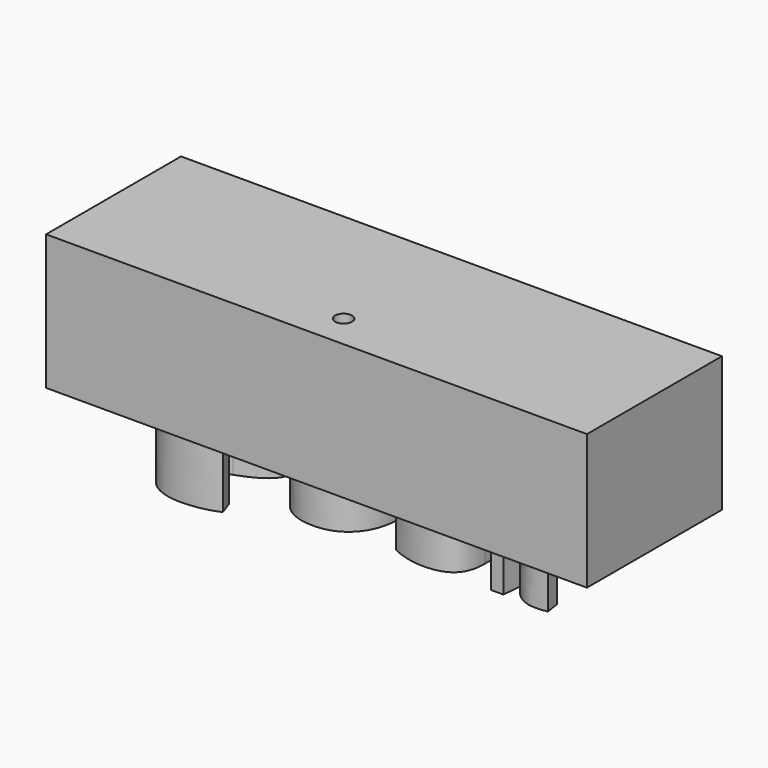
from build123d import *

# Parameters (mm, degrees)
F0_W         = 101.6
F0_H         = 31.6853369992
F1_DEPTH     = 12.7
F3_DEPTH     = 12.7
F5_DEPTH     = 59.182
F2_TEXT_SIZE = 35.1481081081
F6_DEPTH     = 12.7


# Not quite as in the source:
# - Text() gives the source's letters only with a copy of the font that has no kerning and outlines rounded to 1/6400 em; it was checked with that copy


with BuildPart() as f1:
    # F0 (on Top) → F1 (new body)
    with BuildSketch(Plane.XY):
        Rectangle(F0_W, F0_H)
    extrude(amount=F1_DEPTH)

    # F3 (add): a face of the model
    f3_faces = [f1.faces().sort_by_distance(p)[0] for p in [
        (0, 0, 12.7),
    ]]
    extrude(f3_faces, amount=F3_DEPTH)

    # F4 (on face) → F5 (cut)
    with BuildSketch(Plane.XY.offset(25.4)):
        with BuildLine():
            ThreePointArc((0, -11.0801684996), (1.1225320151, -10.6152005147), (1.5875, -9.4926684996))
            ThreePointArc((1.5875, -9.4926684996), (-1.1225320151, -8.3701364845), (0, -11.0801684996))
        make_face()
    extrude(amount=-F5_DEPTH, mode=Mode.SUBTRACT)

    # F2 (on face) → F6 (join)
    with BuildSketch(Plane(origin=(0, 0, 0), x_dir=(1, 0, 0), z_dir=(0, 0, -1))):
        with Locations((-38.1, -12.6533189189)):
            Text('Soar', F2_TEXT_SIZE, font='Open Sans', text_align=(TextAlign.LEFT, TextAlign.BOTTOM))
    extrude(amount=F6_DEPTH)


solid = f1.part
